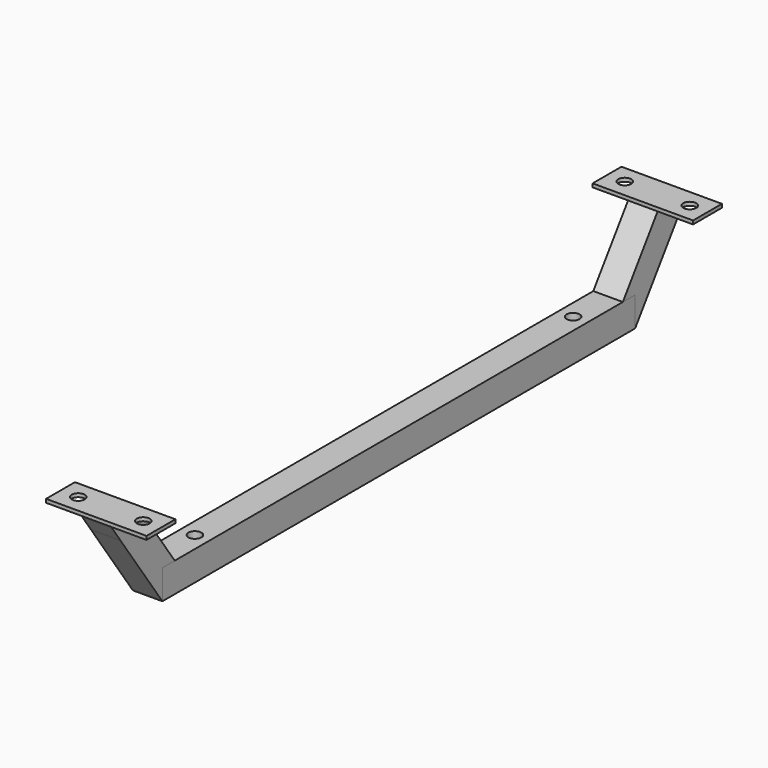
from build123d import *

# Parameters (mm, degrees)
F0_W     = 25
F0_H     = 500
F0_R     = 5.5
F1_DEPTH = 25
F3_DEPTH = 25
F4_W     = 30
F4_H     = 30.519364719
F4_R     = 5.5
F4_W_2   = 25
F5_DEPTH = 3
F4_W_3   = 85


# Not quite as in the source:
# - a feature names something its author has since deleted; it is built from what else it names


with BuildPart() as f1:
    # F0 (on Top) → F1 (new body)
    with BuildSketch(Plane.XY):
        Rectangle(F0_W, F0_H)
        with Locations((0, -200)):
            Circle(F0_R, mode=Mode.SUBTRACT)
        with Locations((0, 200)):
            Circle(F0_R, mode=Mode.SUBTRACT)
    extrude(amount=F1_DEPTH)


with BuildPart() as f3:
    # F2 (on face) → F3 (new body)
    with BuildSketch(Plane.YZ.offset(12.5)):
        Polygon((-294.2501667927, 63.1957875029), (-250, 0), (-250, 25), (-236.9858237362, 25), (-273.7713656854, 77.5351984117), align=None)
        Polygon((-304.2907304045, 77.5351984117), (-294.2501667927, 63.1957875029), (-273.7713656854, 77.5351984117), align=None)
    extrude(amount=-F3_DEPTH)

    # F4 (on face) → F5 (join)
    with BuildSketch(Plane.XY.offset(77.5351984117)):
        with Locations((-27.5, -289.0310480449)):
            Rectangle(F4_W, F4_H)
        with Locations((-27.5, -289.0310480449)):
            Circle(F4_R, mode=Mode.SUBTRACT)
        with Locations((0, -289.0310480449)):
            Rectangle(F4_W_2, F4_H)
        with Locations((27.5, -289.0310480449)):
            Rectangle(F4_W, F4_H)
        with Locations((27.5, -289.0310480449)):
            Circle(F4_R, mode=Mode.SUBTRACT)
    extrude(amount=F5_DEPTH)


with BuildPart() as f3b:
    # F2 (on face) → F3, piece 2 (new body)
    with BuildSketch(Plane.YZ.offset(12.5)):
        Polygon((250, 25), (250, 0), (294.2501667927, 63.1957875029), (273.7713656854, 77.5351984117), (236.9858237362, 25), align=None)
        Polygon((273.7713656854, 77.5351984117), (294.2501667927, 63.1957875029), (304.2907304045, 77.5351984117), align=None)
    extrude(amount=-F3_DEPTH)


with BuildPart() as f5:
    # F4 (on face) → F5, piece 2 (new body)
    with BuildSketch(Plane.XY.offset(77.5351984117)):
        with Locations((0, 289.0310480449)):
            Rectangle(F4_W_3, F4_H)
        with Locations((-27.5, 289.0310480449)):
            Circle(F4_R, mode=Mode.SUBTRACT)
        with Locations((27.5, 289.0310480449)):
            Circle(F4_R, mode=Mode.SUBTRACT)
    extrude(amount=F5_DEPTH)


solid = Compound([f1.part, f3.part, f3b.part, f5.part])
